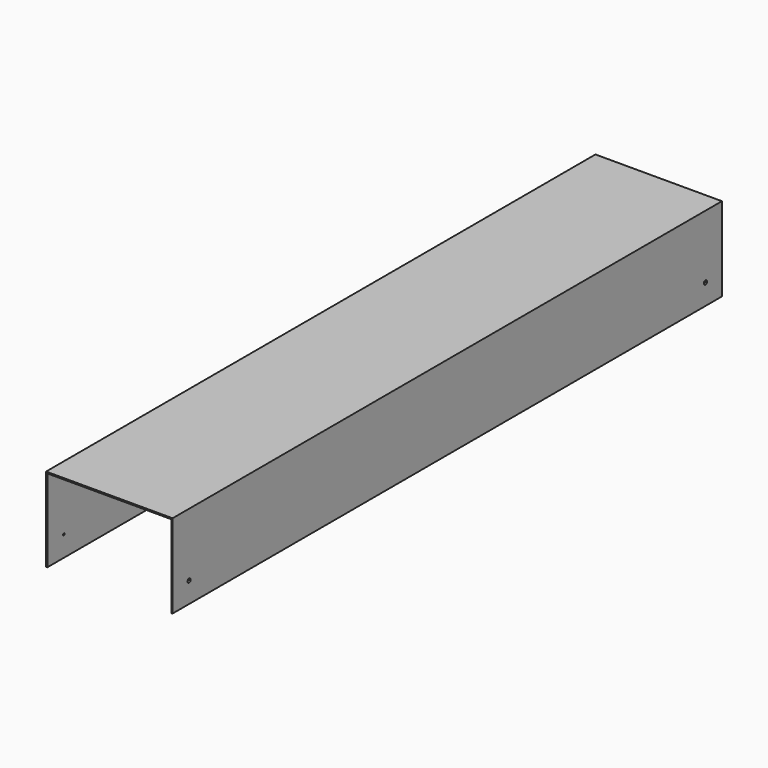
from build123d import *

# Parameters (mm, degrees)
F1_DEPTH         = 844.55
F3_D             = 4.7625
F3_DEPTH         = 25.4
F3_CSINK_D       = 9.525
F3_CSINK_ANGLE   = 90
F3_TIP           = 1.4307993491
F3_COPIES2_COUNT = 2


# Not quite as in the source:
# - a pattern or mirror of a feature is missing from the dataset's text; its kind, count and spacing are read off the source's solid


with BuildPart() as f1:
    # F0 (on Front) → F1 (new body, symmetric)
    with BuildSketch(Plane.XZ):
        Polygon((155.575, -103.1875), (155.575, 103.1875), (-155.575, 103.1875), (-155.575, -103.1875), (-152.4, -103.1875), (-152.4, 100.0125), (152.4, 100.0125), (152.4, -103.1875), align=None)
    extrude(amount=F1_DEPTH, both=True)

    # F3
    with Locations(Plane.YZ.offset(155.575)):
        with Locations((-793.75, -52.3875)):
            f3 = CounterSinkHole(F3_D / 2, F3_CSINK_D / 2, depth=F3_DEPTH, counter_sink_angle=F3_CSINK_ANGLE)
            with Locations((0, 0, -(F3_DEPTH + F3_TIP / 2))):  # 118° drill point
                Cone(0, F3_D / 2, F3_TIP, mode=Mode.SUBTRACT)

    # F3_copies: F3 across plane
    add(f3.mirror(Plane(origin=(0, 0, 0), x_dir=(0, 0, -1), z_dir=(-1, 0, 0))), mode=Mode.SUBTRACT)

    # F3_copies1: F3 across plane
    add(f3.mirror(Plane.ZX), mode=Mode.SUBTRACT)

    # F3_copies2: F3 ×2 about axis
    f3_copies2_axis = Axis((0, 0, 0), (0, 0, 1))
    for i in range(1, F3_COPIES2_COUNT):
        add(f3.rotate(f3_copies2_axis, i * 360 / F3_COPIES2_COUNT), mode=Mode.SUBTRACT)


solid = f1.part
